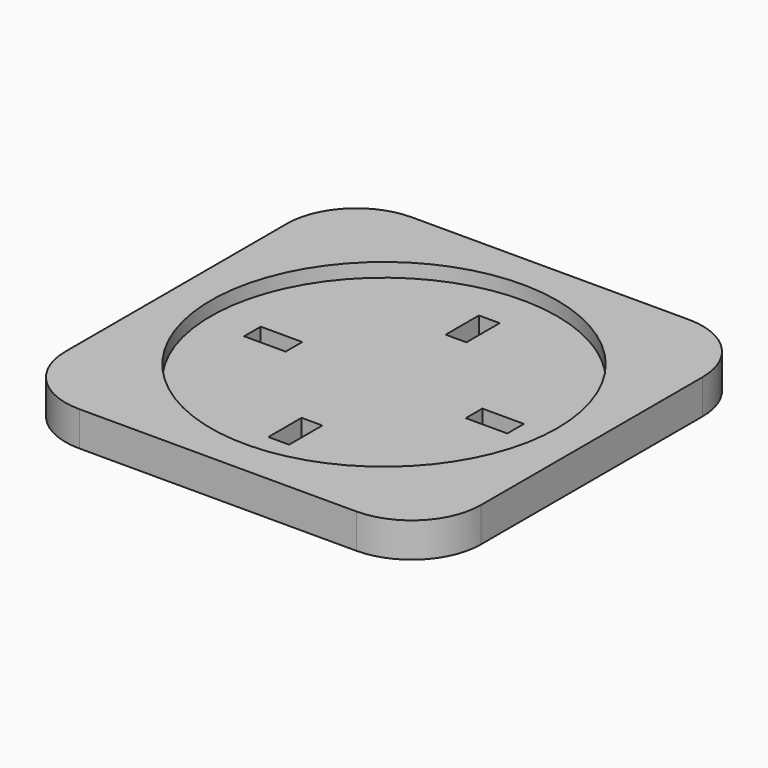
from build123d import *

# Parameters (mm, degrees)
F0_W            = 60
F0_H            = 60
F1_DEPTH        = 5
F2_R            = 10
F3_R            = 25
F4_DEPTH        = 2
F5_W            = 3
F5_H            = 6
F6_DEPTH        = 3
F6_COPIES_COUNT = 4


# Not quite as in the source:
# - a pattern or mirror of a feature is missing from the dataset's text; its kind, count and spacing are read off the source's solid
# - a feature names something its author has since deleted; it is built from what else it names


with BuildPart() as f1:
    # F0 (on Top) → F1 (new body)
    with BuildSketch(Plane.XY):
        Rectangle(F0_W, F0_H)
    extrude(amount=F1_DEPTH)

    # F2
    f2_edges = [f1.edges().sort_by_distance(p)[0] for p in [
        (-30, 30, 2.5),
        (-30, -30, 2.5),
        (30, 30, 2.5),
        (30, -30, 2.5),
    ]]
    fillet(f2_edges, radius=F2_R)

    # F3 (on face) → F4 (cut)
    with BuildSketch(Plane.XY.offset(5)):
        Circle(F3_R)
    extrude(amount=-F4_DEPTH, mode=Mode.SUBTRACT)

    # F5 (on face) → F6 (cut)
    with BuildSketch(Plane.XY.offset(3)):
        with Locations((0, 16)):
            Rectangle(F5_W, F5_H)
    f6 = extrude(amount=-F6_DEPTH, mode=Mode.SUBTRACT)

    # F6_copies: F6 ×4 about axis
    f6_copies_axis = Axis((0, 0, 0), (0, 0, 1))
    for i in range(1, F6_COPIES_COUNT):
        add(f6.rotate(f6_copies_axis, i * 360 / F6_COPIES_COUNT), mode=Mode.SUBTRACT)


solid = f1.part
